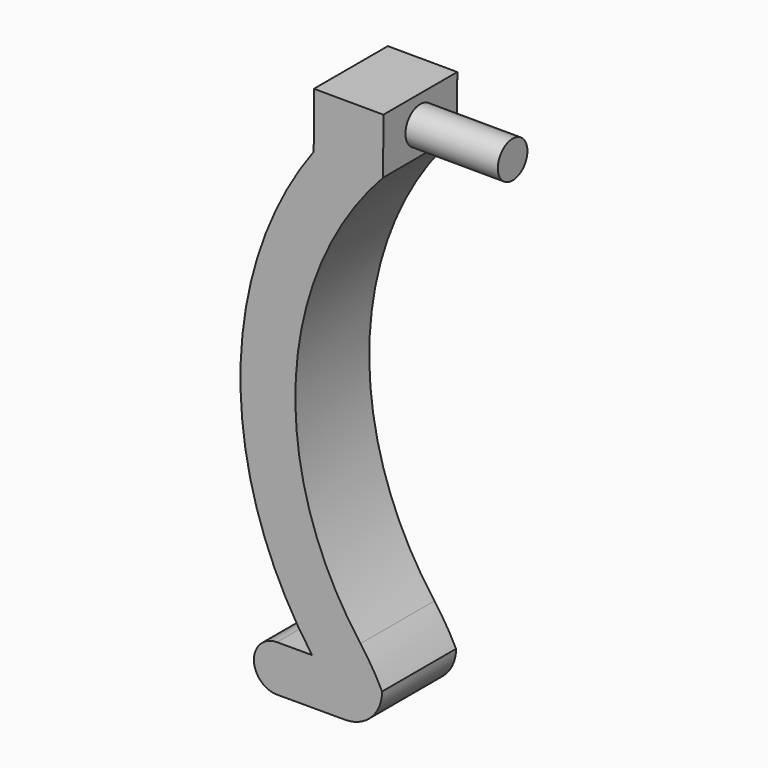
from build123d import *

# Parameters (mm, degrees)
F1_DEPTH    = 12.7
F2_W        = 9.5430067153
F2_H        = 12.7
F3_DEPTH    = 7.62
F4_R        = 2.54
F5_DEPTH    = 12.7
F6_R        = 5.08
F7_T1_DEPTH = 35.8885048544


# Not quite as in the source:
# - a fillet or chamfer that OpenCascade refuses, or shapes differently, is made with other operations: its cross-section is extruded or revolved along the edge and cut away or added


with BuildPart() as f1:
    # F0 (on Front) → F1 (new body)
    with BuildSketch(Plane.XZ):
        with BuildLine():
            Line((-21.0839635167, 28.5975757856), (-30.6269058684, 28.632624914))
            ThreePointArc((-30.6269058684, 28.632624914), (-40.6992100974, -1.826971115), (-30.8592707303, -32.3624242144))
            Line((-30.8592707303, -32.3624242144), (-21.2263563985, -32.3624242144))
            ThreePointArc((-21.2263563985, -32.3624242144), (-33.1531180249, -1.8543988892), (-21.0839635167, 28.5975757856))
        make_face()
        Polygon((-21.2263563985, -32.3624242144), (-30.8592707303, -32.3624242144), (-35.6757278961, -32.3624242144), (-35.6757278961, -38.7124242144), (-21.2263563985, -38.7124242144), align=None)
        with BuildLine():
            Line((-35.6757278961, -38.7124242144), (-35.6757278961, -32.3624242144))
            ThreePointArc((-35.6757278961, -32.3624242144), (-38.8507278961, -35.5374242144), (-35.6757278961, -38.7124242144))
        make_face()
    extrude(amount=F1_DEPTH)

    # F2 (on face) → F3 (join)
    with BuildSketch(Plane(origin=(0.1047467849, 0, 28.519754313), x_dir=(0.9999932554, 0, -0.0036727553), z_dir=(0.0036727553, 0, 0.9999932554))):
        with Locations((-25.9603565693, -6.35)):
            Rectangle(F2_W, F2_H)
    extrude(amount=F3_DEPTH)

    # F4 (on face) → F5 (join)
    with BuildSketch(Plane(origin=(-21.1887103016, 0, 0.0778214726), x_dir=(0, 1, 0), z_dir=(0.9999932554, 0, -0.0036727553))):
        with Locations((-6.35, 32.2985388339)):
            Circle(F4_R)
    extrude(amount=F5_DEPTH)

    # F6
    f6_edges = [f1.edges().sort_by_distance(p)[0] for p in [
        (-21.226356, -6.35, -38.712424),
    ]]
    fillet(f6_edges, radius=F6_R)

    # F7: fillet of radius 30.8120471725 on 1 edges, made by hand

    # F7_s2 → F7_t1 (cut)
    with BuildSketch(Plane.XZ.offset(-11.5942524272)):
        with BuildLine():
            ThreePointArc((-21.2263563985, -33.6324242144), (-22.6013772134, -31.1490637357), (-24.1991044236, -28.8027838569))
            ThreePointArc((-24.1991044236, -28.8027838569), (-22.7589105371, -30.6211702571), (-21.2263563985, -32.3624242144))
            Line((-21.2263563985, -32.3624242144), (-21.2263563985, -33.6324242144))
        make_face()
    extrude(amount=F7_T1_DEPTH, mode=Mode.SUBTRACT)


solid = f1.part
